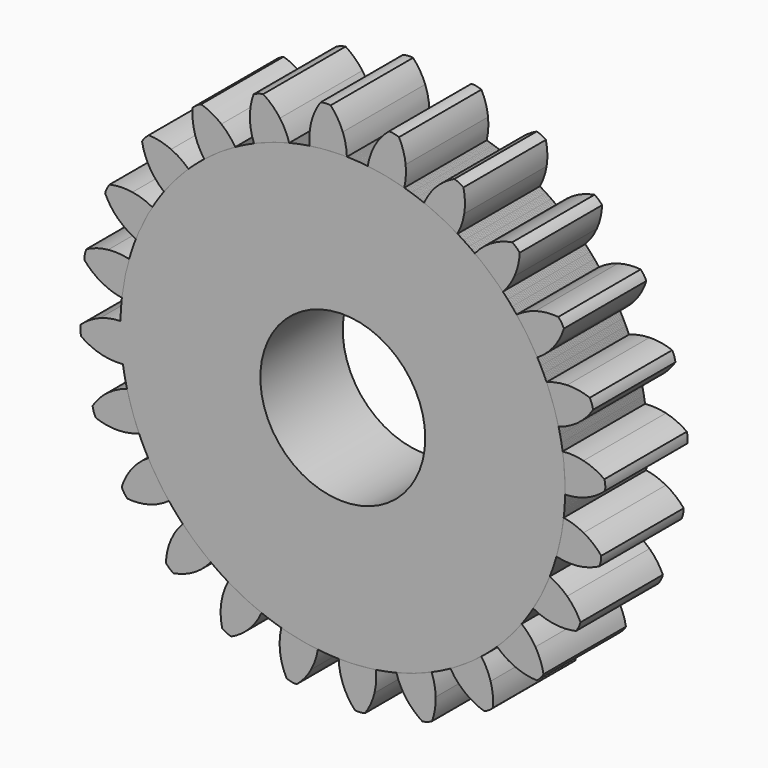
from build123d import *

# Parameters (mm, degrees)
F1_DEPTH = 2.94
F2_COUNT = 24
F3_R     = 2.35294
F4_DEPTH = 2.94
F5_SCALE = 1.7


with BuildPart() as f1:
    # F0 (on Front) → F1 (new body)
    with BuildSketch(Plane.XZ):
        with BuildLine():
            ThreePointArc((-0.9435656978, 6.2744488821), (-4.1395712729, -4.8086354277), (6.345, 0))
            ThreePointArc((6.345, 0), (4.5275988552, 4.4452079374), (0.1165134416, 6.3439301397))
            ThreePointArc((0.1165134416, 6.3439301397), (-0.414982855, 6.3314148679), (-0.9435656978, 6.2744488821))
        make_face()
        with BuildLine():
            ThreePointArc((-0.9435656978, 6.2744488821), (-0.414982855, 6.3314148679), (0.1165134416, 6.3439301397))
            ThreePointArc((0.1165134416, 6.3439301397), (0.0834300033, 6.6419696367), (0, 6.93))
            ThreePointArc((0, 6.93), (-0.1465929508, 7.2243794205), (-0.3458241883, 7.4860197279))
            ThreePointArc((-0.3458241883, 7.4860197279), (-0.4909334511, 7.4901970386), (-0.6342560355, 7.4671149059))
            ThreePointArc((-0.6342560355, 7.4671149059), (-0.7976319091, 7.1817080728), (-0.9045465121, 6.8707128893))
            ThreePointArc((-0.9045465121, 6.8707128893), (-0.9496672536, 6.5742568651), (-0.9435656978, 6.2744488821))
        make_face()
    extrude(amount=F1_DEPTH)


with BuildPart() as f2_1:
    # F2: instance of F1
    add(f1.part.rotate(Axis((0, 0, 0), (0, 1, 0)), 1 * 360 / F2_COUNT))


with BuildPart() as f2_2:
    # F2: instance of F1
    add(f1.part.rotate(Axis((0, 0, 0), (0, 1, 0)), 2 * 360 / F2_COUNT))


with BuildPart() as f2_3:
    # F2: instance of F1
    add(f1.part.rotate(Axis((0, 0, 0), (0, 1, 0)), 3 * 360 / F2_COUNT))


with BuildPart() as f2_4:
    # F2: instance of F1
    add(f1.part.rotate(Axis((0, 0, 0), (0, 1, 0)), 4 * 360 / F2_COUNT))


with BuildPart() as f2_5:
    # F2: instance of F1
    add(f1.part.rotate(Axis((0, 0, 0), (0, 1, 0)), 5 * 360 / F2_COUNT))


with BuildPart() as f2_6:
    # F2: instance of F1
    add(f1.part.rotate(Axis((0, 0, 0), (0, 1, 0)), 6 * 360 / F2_COUNT))


with BuildPart() as f2_7:
    # F2: instance of F1
    add(f1.part.rotate(Axis((0, 0, 0), (0, 1, 0)), 7 * 360 / F2_COUNT))


with BuildPart() as f2_8:
    # F2: instance of F1
    add(f1.part.rotate(Axis((0, 0, 0), (0, 1, 0)), 8 * 360 / F2_COUNT))


with BuildPart() as f2_9:
    # F2: instance of F1
    add(f1.part.rotate(Axis((0, 0, 0), (0, 1, 0)), 9 * 360 / F2_COUNT))


with BuildPart() as f2_10:
    # F2: instance of F1
    add(f1.part.rotate(Axis((0, 0, 0), (0, 1, 0)), 10 * 360 / F2_COUNT))


with BuildPart() as f2_11:
    # F2: instance of F1
    add(f1.part.rotate(Axis((0, 0, 0), (0, 1, 0)), 11 * 360 / F2_COUNT))


with BuildPart() as f2_12:
    # F2: instance of F1
    add(f1.part.rotate(Axis((0, 0, 0), (0, 1, 0)), 12 * 360 / F2_COUNT))


with BuildPart() as f2_13:
    # F2: instance of F1
    add(f1.part.rotate(Axis((0, 0, 0), (0, 1, 0)), 13 * 360 / F2_COUNT))


with BuildPart() as f2_14:
    # F2: instance of F1
    add(f1.part.rotate(Axis((0, 0, 0), (0, 1, 0)), 14 * 360 / F2_COUNT))


with BuildPart() as f2_15:
    # F2: instance of F1
    add(f1.part.rotate(Axis((0, 0, 0), (0, 1, 0)), 15 * 360 / F2_COUNT))


with BuildPart() as f2_16:
    # F2: instance of F1
    add(f1.part.rotate(Axis((0, 0, 0), (0, 1, 0)), 16 * 360 / F2_COUNT))


with BuildPart() as f2_17:
    # F2: instance of F1
    add(f1.part.rotate(Axis((0, 0, 0), (0, 1, 0)), 17 * 360 / F2_COUNT))


with BuildPart() as f2_18:
    # F2: instance of F1
    add(f1.part.rotate(Axis((0, 0, 0), (0, 1, 0)), 18 * 360 / F2_COUNT))


with BuildPart() as f2_19:
    # F2: instance of F1
    add(f1.part.rotate(Axis((0, 0, 0), (0, 1, 0)), 19 * 360 / F2_COUNT))


with BuildPart() as f2_20:
    # F2: instance of F1
    add(f1.part.rotate(Axis((0, 0, 0), (0, 1, 0)), 20 * 360 / F2_COUNT))


with BuildPart() as f2_21:
    # F2: instance of F1
    add(f1.part.rotate(Axis((0, 0, 0), (0, 1, 0)), 21 * 360 / F2_COUNT))


with BuildPart() as f2_22:
    # F2: instance of F1
    add(f1.part.rotate(Axis((0, 0, 0), (0, 1, 0)), 22 * 360 / F2_COUNT))


with BuildPart() as f2_23:
    # F2: instance of F1
    add(f1.part.rotate(Axis((0, 0, 0), (0, 1, 0)), 23 * 360 / F2_COUNT))


with BuildPart() as f4_tool:
    # F3 (on face) → F4 (new body, through all)
    with BuildSketch(Plane.XZ.offset(2.94)):
        Circle(F3_R)
    extrude(amount=-F4_DEPTH)


with BuildPart() as f1_1:
    add(f1.part)

    # F4: cut by f4_tool
    add(f4_tool.part, mode=Mode.SUBTRACT)


with BuildPart() as f2_1_1:
    add(f2_1.part)

    # F4: cut by f4_tool
    add(f4_tool.part, mode=Mode.SUBTRACT)


with BuildPart() as f2_2_1:
    add(f2_2.part)

    # F4: cut by f4_tool
    add(f4_tool.part, mode=Mode.SUBTRACT)


with BuildPart() as f2_3_1:
    add(f2_3.part)

    # F4: cut by f4_tool
    add(f4_tool.part, mode=Mode.SUBTRACT)


with BuildPart() as f2_4_1:
    add(f2_4.part)

    # F4: cut by f4_tool
    add(f4_tool.part, mode=Mode.SUBTRACT)


with BuildPart() as f2_5_1:
    add(f2_5.part)

    # F4: cut by f4_tool
    add(f4_tool.part, mode=Mode.SUBTRACT)


with BuildPart() as f2_6_1:
    add(f2_6.part)

    # F4: cut by f4_tool
    add(f4_tool.part, mode=Mode.SUBTRACT)


with BuildPart() as f2_7_1:
    add(f2_7.part)

    # F4: cut by f4_tool
    add(f4_tool.part, mode=Mode.SUBTRACT)


with BuildPart() as f2_8_1:
    add(f2_8.part)

    # F4: cut by f4_tool
    add(f4_tool.part, mode=Mode.SUBTRACT)


with BuildPart() as f2_9_1:
    add(f2_9.part)

    # F4: cut by f4_tool
    add(f4_tool.part, mode=Mode.SUBTRACT)


with BuildPart() as f2_10_1:
    add(f2_10.part)

    # F4: cut by f4_tool
    add(f4_tool.part, mode=Mode.SUBTRACT)


with BuildPart() as f2_11_1:
    add(f2_11.part)

    # F4: cut by f4_tool
    add(f4_tool.part, mode=Mode.SUBTRACT)


with BuildPart() as f2_12_1:
    add(f2_12.part)

    # F4: cut by f4_tool
    add(f4_tool.part, mode=Mode.SUBTRACT)


with BuildPart() as f2_13_1:
    add(f2_13.part)

    # F4: cut by f4_tool
    add(f4_tool.part, mode=Mode.SUBTRACT)


with BuildPart() as f2_14_1:
    add(f2_14.part)

    # F4: cut by f4_tool
    add(f4_tool.part, mode=Mode.SUBTRACT)


with BuildPart() as f2_15_1:
    add(f2_15.part)

    # F4: cut by f4_tool
    add(f4_tool.part, mode=Mode.SUBTRACT)


with BuildPart() as f2_16_1:
    add(f2_16.part)

    # F4: cut by f4_tool
    add(f4_tool.part, mode=Mode.SUBTRACT)


with BuildPart() as f2_17_1:
    add(f2_17.part)

    # F4: cut by f4_tool
    add(f4_tool.part, mode=Mode.SUBTRACT)


with BuildPart() as f2_18_1:
    add(f2_18.part)

    # F4: cut by f4_tool
    add(f4_tool.part, mode=Mode.SUBTRACT)


with BuildPart() as f2_19_1:
    add(f2_19.part)

    # F4: cut by f4_tool
    add(f4_tool.part, mode=Mode.SUBTRACT)


with BuildPart() as f2_20_1:
    add(f2_20.part)

    # F4: cut by f4_tool
    add(f4_tool.part, mode=Mode.SUBTRACT)


with BuildPart() as f2_21_1:
    add(f2_21.part)

    # F4: cut by f4_tool
    add(f4_tool.part, mode=Mode.SUBTRACT)


with BuildPart() as f2_22_1:
    add(f2_22.part)

    # F4: cut by f4_tool
    add(f4_tool.part, mode=Mode.SUBTRACT)


with BuildPart() as f2_23_1:
    add(f2_23.part)

    # F4: cut by f4_tool
    add(f4_tool.part, mode=Mode.SUBTRACT)


with BuildPart() as f2_23_2:
    # F5: moved
    add(f2_23_1.part.scale(F5_SCALE))


with BuildPart() as f2_11_2:
    # F5: moved
    add(f2_11_1.part.scale(F5_SCALE))


with BuildPart() as f2_12_2:
    # F5: moved
    add(f2_12_1.part.scale(F5_SCALE))


with BuildPart() as f2_3_2:
    # F5: moved
    add(f2_3_1.part.scale(F5_SCALE))


with BuildPart() as f2_13_2:
    # F5: moved
    add(f2_13_1.part.scale(F5_SCALE))


with BuildPart() as f2_7_2:
    # F5: moved
    add(f2_7_1.part.scale(F5_SCALE))


with BuildPart() as f2_8_2:
    # F5: moved
    add(f2_8_1.part.scale(F5_SCALE))


with BuildPart() as f2_1_2:
    # F5: moved
    add(f2_1_1.part.scale(F5_SCALE))


with BuildPart() as f2_14_2:
    # F5: moved
    add(f2_14_1.part.scale(F5_SCALE))


with BuildPart() as f2_21_2:
    # F5: moved
    add(f2_21_1.part.scale(F5_SCALE))


with BuildPart() as f2_9_2:
    # F5: moved
    add(f2_9_1.part.scale(F5_SCALE))


with BuildPart() as f2_2_2:
    # F5: moved
    add(f2_2_1.part.scale(F5_SCALE))


with BuildPart() as f1_2:
    # F5: moved
    add(f1_1.part.scale(F5_SCALE))


with BuildPart() as f2_22_2:
    # F5: moved
    add(f2_22_1.part.scale(F5_SCALE))


with BuildPart() as f2_4_2:
    # F5: moved
    add(f2_4_1.part.scale(F5_SCALE))


with BuildPart() as f2_16_2:
    # F5: moved
    add(f2_16_1.part.scale(F5_SCALE))


with BuildPart() as f2_10_2:
    # F5: moved
    add(f2_10_1.part.scale(F5_SCALE))


with BuildPart() as f2_17_2:
    # F5: moved
    add(f2_17_1.part.scale(F5_SCALE))


with BuildPart() as f2_15_2:
    # F5: moved
    add(f2_15_1.part.scale(F5_SCALE))


with BuildPart() as f2_5_2:
    # F5: moved
    add(f2_5_1.part.scale(F5_SCALE))


with BuildPart() as f2_6_2:
    # F5: moved
    add(f2_6_1.part.scale(F5_SCALE))


with BuildPart() as f2_20_2:
    # F5: moved
    add(f2_20_1.part.scale(F5_SCALE))


with BuildPart() as f2_19_2:
    # F5: moved
    add(f2_19_1.part.scale(F5_SCALE))


with BuildPart() as f2_18_2:
    # F5: moved
    add(f2_18_1.part.scale(F5_SCALE))


solid = Compound([f2_23_2.part, f2_11_2.part, f2_12_2.part, f2_3_2.part, f2_13_2.part, f2_7_2.part, f2_8_2.part, f2_1_2.part, f2_14_2.part, f2_21_2.part, f2_9_2.part, f2_2_2.part, f1_2.part, f2_22_2.part, f2_4_2.part, f2_16_2.part, f2_10_2.part, f2_17_2.part, f2_15_2.part, f2_5_2.part, f2_6_2.part, f2_20_2.part, f2_19_2.part, f2_18_2.part])
